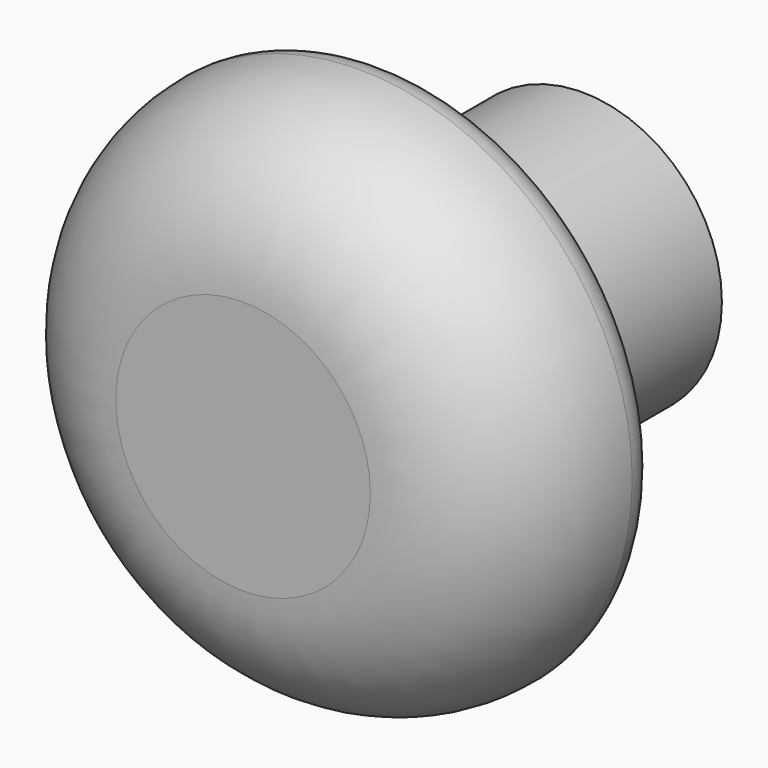
from build123d import *

# Parameters (mm, degrees)
F0_R     = 11.5
F0_R_2   = 10.25
F1_DEPTH = 20
F2_R     = 22.5
F3_DEPTH = 15
F4_R     = 12
F5_R     = 2.99999


# Not quite as in the source:
# - a fillet or chamfer is up to 0.001 mm smaller than in the source, because OpenCascade refuses the exact size


with BuildPart() as f1:
    # F0 (on Front) → F1 (new body)
    with BuildSketch(Plane.XZ):
        Circle(F0_R)
        Circle(F0_R_2, mode=Mode.SUBTRACT)
    extrude(amount=F1_DEPTH)

    # F2 (on face) → F3 (join)
    with BuildSketch(Plane.XZ.offset(20)):
        Circle(F2_R)
    extrude(amount=F3_DEPTH)

    # F4
    f4_edges = [f1.edges().sort_by_distance(p)[0] for p in [
        (-22.5, -35, 0),
    ]]
    fillet(f4_edges, radius=F4_R)

    # F5 (radius 3 in the source; OpenCascade refuses exactly that, so slightly less here)
    f5_edges = [f1.edges().sort_by_distance(p)[0] for p in [
        (-10.5, -35, 0),
        (-22.5, -23, 0),
        (-22.5, -20, 0),
    ]]
    fillet(f5_edges, radius=F5_R)


solid = f1.part
